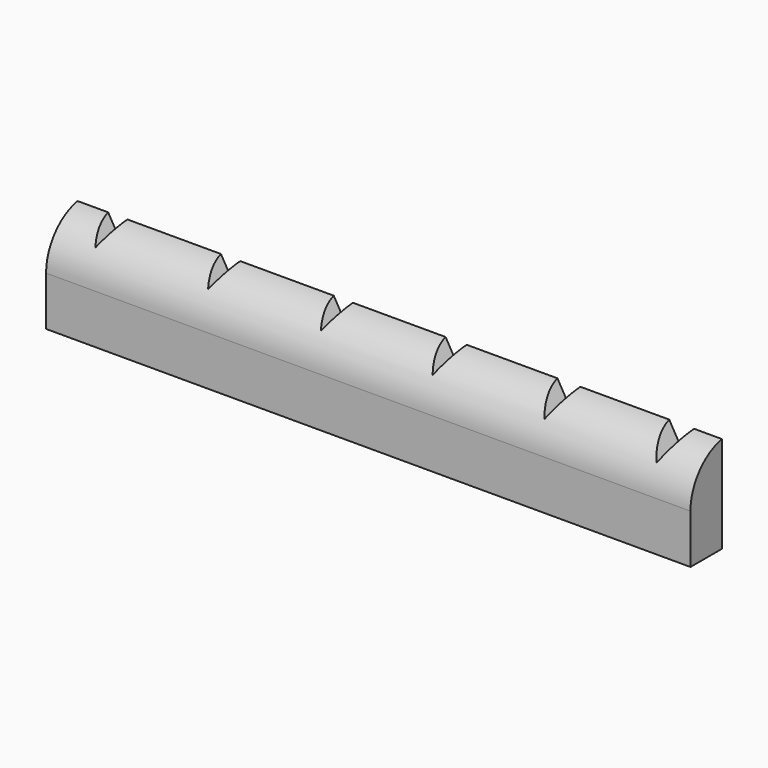
from build123d import *

# Parameters (mm, degrees)
F0_W        = 50.8
F0_H        = 3.0988
F1_DEPTH    = 7.62
F3_T1_DEPTH = 69.5151640121
F4_DEPTH    = 25.4


# Not quite as in the source:
# - a fillet or chamfer that OpenCascade refuses, or shapes differently, is made with other operations: its cross-section is extruded or revolved along the edge and cut away or added


with BuildPart() as f1:
    # F0 (on Top) → F1 (new body)
    with BuildSketch(Plane.XY):
        with Locations((0, 1.5494)):
            Rectangle(F0_W, F0_H)
    extrude(amount=F1_DEPTH)

    # F3: fillet of radius 3.81 on 1 edges, made by hand

    # F3_s2 → F3_t1 (cut)
    with BuildSketch(Plane.YZ.offset(-34.7575820061)):
        with BuildLine():
            ThreePointArc((0, 3.8769671976), (0.8752281179, 6.3066202592), (3.0988, 7.62))
            Line((3.0988, 7.62), (0, 7.62))
            Line((0, 7.62), (0, 3.8769671976))
        make_face()
    extrude(amount=F3_T1_DEPTH, mode=Mode.SUBTRACT)

    # F2 (on face) → F4 (cut)
    with BuildSketch(Plane.XZ):
        Polygon((-22.225, 6.3092954744), (-21.4682643893, 7.62), (-22.9817356107, 7.62), align=None)
        Polygon((-12.5782643893, 7.62), (-14.0917356107, 7.62), (-13.335, 6.3092954744), align=None)
        Polygon((14.2383825791, 7.62), (12.4316174209, 7.62), (13.335, 6.0552954744), align=None)
        Polygon((22.225, 5.9282954744), (23.2017060633, 7.62), (21.2482939367, 7.62), align=None)
        Polygon((-3.6882643893, 7.62), (-5.2017356107, 7.62), (-4.445, 6.3092954744), align=None)
        Polygon((5.2750590949, 7.62), (3.6149409051, 7.62), (4.445, 6.1822954744), align=None)
    extrude(amount=-F4_DEPTH, mode=Mode.SUBTRACT)


solid = f1.part
